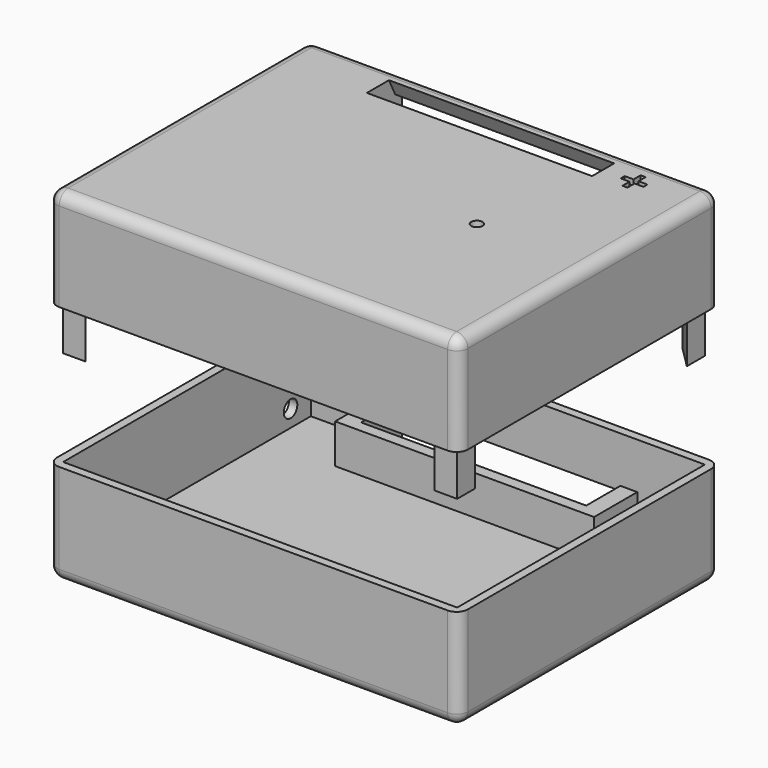
from build123d import *

# Parameters (mm, degrees)
F0_W          = 70
F0_H          = 55
F1_DEPTH      = 2.8
F2_DEPTH      = 18
F4_DEPTH      = 7
F3_W          = 40
F3_H          = 6.3
F5_W          = 40
F5_H          = 4.9
F7_W          = 40
F7_H          = 6.2
F8_DEPTH      = 1.5
F9_R          = 1.5
F10_DEPTH     = 1.5
F11_R         = 2
F12_TEXT_SIZE = 8.9411520296
F13_DEPTH     = 1
F16_DEPTH     = 15
F18_DEPTH     = 2.8
F19_W         = 40
F19_H         = 6.3
F20_W         = 40
F20_H         = 4.9
F22_DEPTH     = 7
F23_W         = 40
F23_H         = 6.2
F24_DEPTH     = 1.5
F25_TEXT_SIZE = 8.3333333333
F26_DEPTH     = 1
F27_R         = 2
F28_R         = 1
F29_DEPTH     = 2.8
F30_R         = 5.25
F30_R_2       = 1
F31_DEPTH     = 1
F32_DEPTH     = 8


# Not quite as in the source:
# - Text() gives the source's letters only with a copy of the font that has no kerning and outlines rounded to 1/6400 em; it was checked with that copy


with BuildPart() as f1:
    # F0 (on Top) → F1 (new body)
    with BuildSketch(Plane.XY):
        with Locations((35, 27.5)):
            Rectangle(F0_W, F0_H)
    extrude(amount=F1_DEPTH)

    # F0 (on Top) → F2 (join)
    with BuildSketch(Plane.XY):
        with BuildLine():
            Line((69.5, 56.5), (0.5, 56.5))
            ThreePointArc((0.5, 56.5), (-0.9142135624, 55.9142135624), (-1.5, 54.5))
            Line((-1.5, 54.5), (-1.5, 0.5))
            ThreePointArc((-1.5, 0.5), (-0.9142135624, -0.9142135624), (0.5, -1.5))
            Line((0.5, -1.5), (69.5, -1.5))
            ThreePointArc((69.5, -1.5), (70.9142135624, -0.9142135624), (71.5, 0.5))
            Line((71.5, 0.5), (71.5, 54.5))
            ThreePointArc((71.5, 54.5), (70.9142135624, 55.9142135624), (69.5, 56.5))
        make_face()
        with Locations((35, 27.5)):
            Rectangle(F0_W, F0_H, mode=Mode.SUBTRACT)
    extrude(amount=F2_DEPTH)

    # F3 (on face) → F4 (join)
    with BuildSketch(Plane.XY.offset(2.8)):
        Polygon((15, 55), (12, 55), (12, 45.4), (58, 45.4), (58, 55), (55, 55), (55, 48.7), (55, 47.4), (15, 47.4), (15, 48.7), align=None)
    extrude(amount=F4_DEPTH)

    # F3 (on face) → F6 section 0
    with BuildSketch(Plane.XY.offset(2.8)):
        with Locations((35, 51.85)):
            Rectangle(F3_W, F3_H)
    # F5 (on face) → F6 section 1
    with BuildSketch(Plane(origin=(0, 0, 0), x_dir=(1, 0, 0), z_dir=(0, 0, -1))):
        with Locations((35, -51.15)):
            Rectangle(F5_W, F5_H)
    loft(mode=Mode.SUBTRACT)

    # F7 (on face) → F8 (cut, through all)
    with BuildSketch(Plane.XZ.offset(-55)):
        with Locations((35, 5.9)):
            Rectangle(F7_W, F7_H)
    extrude(amount=-F8_DEPTH, mode=Mode.SUBTRACT)

    # F9 (on face) → F10 (cut, through all)
    with BuildSketch(Plane(origin=(-1.5, 0, 0), x_dir=(0, -1, 0), z_dir=(-1, 0, 0))):
        with Locations((-50.5, 5.8)):
            Circle(F9_R)
    extrude(amount=-F10_DEPTH, mode=Mode.SUBTRACT)

    # F11
    f11_edges = [f1.edges().sort_by_distance(p)[0] for p in [
        (35, -1.5, 0),
    ]]
    fillet(f11_edges, radius=F11_R)

    # F12 (on face) → F13 (cut)
    with BuildSketch(Plane(origin=(0, 0, 0), x_dir=(1, 0, 0), z_dir=(0, 0, -1))):
        with Locations((57.5964790769, -53.2253757119)):
            Text('-', F12_TEXT_SIZE, font='Open Sans', font_style=FontStyle.BOLD, text_align=(TextAlign.LEFT, TextAlign.BOTTOM))
    extrude(amount=-F13_DEPTH, mode=Mode.SUBTRACT)


with BuildPart() as f16:
    # F15 (on offset) → F16 (new body)
    with BuildSketch(Plane.XY.offset(43)):
        with BuildLine():
            Line((69.5, 56.5), (0.5, 56.5))
            ThreePointArc((0.5, 56.5), (-0.9142135624, 55.9142135624), (-1.5, 54.5))
            Line((-1.5, 54.5), (-1.5, 0.5))
            ThreePointArc((-1.5, 0.5), (-0.9142135624, -0.9142135624), (0.5, -1.5))
            Line((0.5, -1.5), (69.5, -1.5))
            ThreePointArc((69.5, -1.5), (70.9142135624, -0.9142135624), (71.5, 0.5))
            Line((71.5, 0.5), (71.5, 54.5))
            ThreePointArc((71.5, 54.5), (70.9142135624, 55.9142135624), (69.5, 56.5))
        make_face()
        Polygon((0, 51), (0, 55), (4, 55), (66, 55), (70, 55), (70, 51), (70, 4), (70, 0), (66, 0), (4, 0), (0, 0), (0, 4), align=None, mode=Mode.SUBTRACT)
        Polygon((4, 0), (0, 4), (0, 0), align=None)
        Polygon((4, 55), (0, 55), (0, 51), align=None)
        Polygon((70, 55), (66, 55), (70, 51), align=None)
        Polygon((70, 0), (70, 4), (66, 0), align=None)
    extrude(amount=F16_DEPTH)

    # F17 (on face) → F18 (join)
    with BuildSketch(Plane.XY.offset(58)):
        with BuildLine():
            Line((69.5, 56.5), (0.5, 56.5))
            ThreePointArc((0.5, 56.5), (-0.9142135624, 55.9142135624), (-1.5, 54.5))
            Line((-1.5, 54.5), (-1.5, 0.5))
            ThreePointArc((-1.5, 0.5), (-0.9142135624, -0.9142135624), (0.5, -1.5))
            Line((0.5, -1.5), (69.5, -1.5))
            ThreePointArc((69.5, -1.5), (70.9142135624, -0.9142135624), (71.5, 0.5))
            Line((71.5, 0.5), (71.5, 54.5))
            ThreePointArc((71.5, 54.5), (70.9142135624, 55.9142135624), (69.5, 56.5))
        make_face()
        Polygon((0, 51), (4, 55), (66, 55), (70, 51), (70, 4), (66, 0), (4, 0), (0, 4), align=None, mode=Mode.SUBTRACT)
        Polygon((66, 55), (4, 55), (0, 51), (0, 4), (4, 0), (66, 0), (70, 4), (70, 51), align=None)
    extrude(amount=F18_DEPTH)

    # F19 (on face) → F21 section 0
    with BuildSketch(Plane(origin=(0, 0, 58), x_dir=(1, 0, 0), z_dir=(0, 0, -1))):
        with Locations((35, -51.85)):
            Rectangle(F19_W, F19_H)
    # F20 (on face) → F21 section 1
    with BuildSketch(Plane.XY.offset(60.8)):
        with Locations((35, 51.15)):
            Rectangle(F20_W, F20_H)
    loft(mode=Mode.SUBTRACT)

    # F19 (on face) → F22 (join)
    with BuildSketch(Plane(origin=(0, 0, 58), x_dir=(1, 0, 0), z_dir=(0, 0, -1))):
        Polygon((12, -45.4), (12, -55), (15, -55), (15, -48.7), (15, -47.4), (55, -47.4), (55, -48.7), (55, -55), (58, -55), (58, -45.4), align=None)
    extrude(amount=F22_DEPTH)

    # F23 (on face) → F24 (cut, through all)
    with BuildSketch(Plane.XZ.offset(-55)):
        with Locations((35, 54.9)):
            Rectangle(F23_W, F23_H)
    extrude(amount=-F24_DEPTH, mode=Mode.SUBTRACT)

    # F25 (on face) → F26 (cut)
    with BuildSketch(Plane.XY.offset(60.8)):
        with Locations((58.1780448556, 48.1430413723)):
            Text('+', F25_TEXT_SIZE, font='Open Sans', font_style=FontStyle.BOLD, text_align=(TextAlign.LEFT, TextAlign.BOTTOM))
    extrude(amount=-F26_DEPTH, mode=Mode.SUBTRACT)

    # F27
    f27_edges = [f16.edges().sort_by_distance(p)[0] for p in [
        (35, -1.5, 60.8),
    ]]
    fillet(f27_edges, radius=F27_R)

    # F28 (on face) → F29 (cut, through all)
    with BuildSketch(Plane.XY.offset(60.8)):
        with Locations((51.5, 27.5)):
            Circle(F28_R)
    extrude(amount=-F29_DEPTH, mode=Mode.SUBTRACT)

    # F30 (on face) → F31 (cut)
    with BuildSketch(Plane(origin=(0, 0, 58), x_dir=(1, 0, 0), z_dir=(0, 0, -1))):
        with Locations((51.5, -27.5)):
            Circle(F30_R)
        with Locations((51.5, -27.5)):
            Circle(F30_R_2, mode=Mode.SUBTRACT)
    extrude(amount=-F31_DEPTH, mode=Mode.SUBTRACT)

    # F15 (on offset) → F32 (join)
    with BuildSketch(Plane.XY.offset(43)):
        Polygon((4, 0), (0, 4), (0, 0), align=None)
        Polygon((70, 0), (70, 4), (66, 0), align=None)
        Polygon((70, 55), (66, 55), (70, 51), align=None)
        Polygon((4, 55), (0, 55), (0, 51), align=None)
    extrude(amount=-F32_DEPTH)


solid = Compound([f1.part, f16.part])
